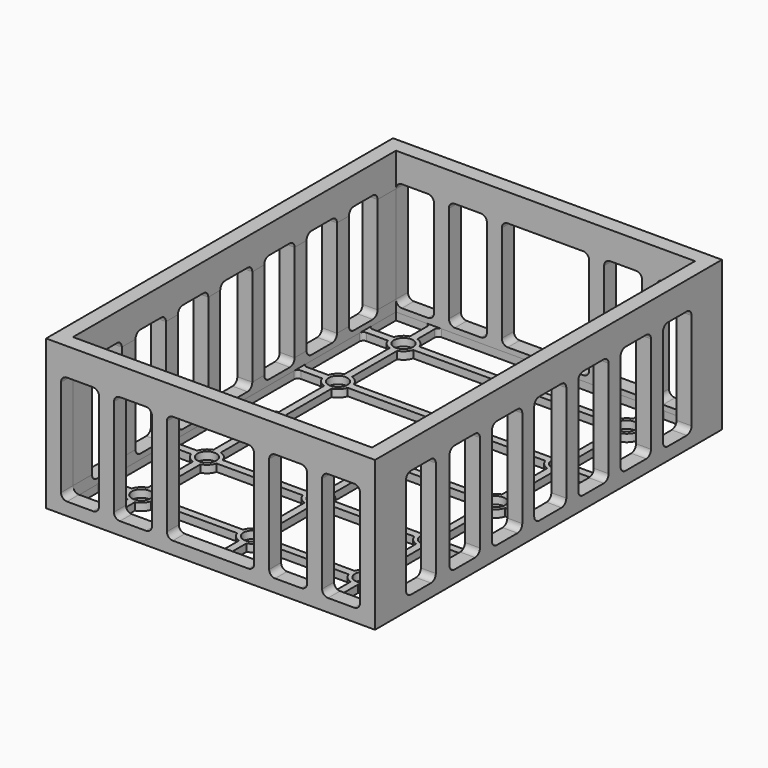
from build123d import *
from build123d import SkipClean  # not in build123d's __all__

# Parameters (mm, degrees)
F0_W      = 440
F0_H      = 580
F1_DEPTH  = 200
F2_W      = 400
F2_H      = 540
F3_DEPTH  = 190
F5_DEPTH  = 10
F4_R      = 12.7
F6_DEPTH  = 10
F8_DEPTH  = 440
F10_DEPTH = 580


# Not quite as in the source:
# - ends of sketch curves that miss each other by under 0.0002 mm in the source are joined


with BuildPart() as f1:
    # F0 (on Top) → F1 (new body)
    with BuildSketch(Plane.XY):
        with Locations((220, 290)):
            Rectangle(F0_W, F0_H)
    extrude(amount=F1_DEPTH)

    # F2 (on face) → F3 (cut)
    with BuildSketch(Plane.XY.offset(200)):
        with Locations((220, 290)):
            Rectangle(F2_W, F2_H)
    extrude(amount=-F3_DEPTH, mode=Mode.SUBTRACT)

    # F4 (on face) → F5 (cut, through all)
    with BuildSketch(Plane.XY.offset(10)):
        with BuildLine():
            ThreePointArc((53.8208951944, 514.2), (58.284209973, 521.715790027), (65.8, 526.1791048056))
            Line((65.8, 526.1791048056), (65.8, 555))
            ThreePointArc((65.8, 555), (64.3355339059, 558.5355339059), (60.8, 560))
            Line((60.8, 560), (20, 560))
            Line((20, 560), (20, 519.2))
            ThreePointArc((20, 519.2), (21.4644660941, 515.6644660941), (25, 514.2))
            Line((25, 514.2), (53.8208951944, 514.2))
        make_face()
        with BuildLine():
            ThreePointArc((75.8000016212, 526.1791043282), (83.3157906245, 521.7157894295), (87.7791048056, 514.2))
            Line((87.7791048056, 514.2), (203.0208951944, 514.2))
            ThreePointArc((203.0208951944, 514.2), (207.484209973, 521.715790027), (215, 526.1791048056))
            Line((215, 526.1791048056), (215, 555))
            ThreePointArc((215, 555), (213.5355339059, 558.5355339059), (210, 560))
            Line((210, 560), (80.8000016212, 560))
            ThreePointArc((80.8000016212, 560), (77.2644677153, 558.5355339059), (75.8000016212, 555))
            Line((75.8000016212, 555), (75.8000016212, 526.1791043282))
        make_face()
        with BuildLine():
            Line((225, 555), (225, 526.1791048056))
            ThreePointArc((225, 526.1791048056), (232.515790027, 521.715790027), (236.9791048056, 514.2))
            Line((236.9791048056, 514.2), (352.22089302, 514.2000006389))
            ThreePointArc((352.22089302, 514.2000006389), (356.684207757, 521.7157906907), (364.1999977593, 526.1791055109))
            Line((364.1999977593, 526.1791055109), (364.1999975996, 555.0000000277))
            ThreePointArc((364.1999975996, 555.0000000277), (362.7355314957, 558.5355339157), (359.1999975996, 560))
            Line((359.1999975996, 560), (230, 560))
            ThreePointArc((230, 560), (226.4644660941, 558.5355339059), (225, 555))
        make_face()
        with BuildLine():
            Line((419.9999978256, 560), (379.1999975996, 560))
            ThreePointArc((379.1999975996, 560), (375.6644636838, 558.5355338961), (374.1999975996, 554.9999999723))
            Line((374.1999975996, 554.9999999723), (374.1999977593, 526.1791055663))
            ThreePointArc((374.1999977593, 526.1791055663), (381.715787811, 521.7157908294), (386.1791026313, 514.2000008271))
            Line((386.1791026313, 514.2000008271), (414.9999978256, 514.2000009868))
            ThreePointArc((414.9999978256, 514.2000009868), (418.5355317316, 515.6644660941), (419.9999978256, 519.2))
            Line((419.9999978256, 519.2), (419.9999978256, 560))
        make_face()
        with BuildLine():
            Line((65.8, 416.5791048056), (65.8, 492.2208951944))
            ThreePointArc((65.8, 492.2208951944), (58.284209973, 496.684209973), (53.8208951944, 504.2))
            Line((53.8208951944, 504.2), (25, 504.2))
            ThreePointArc((25, 504.2), (21.4644660941, 502.7355339059), (20, 499.2))
            Line((20, 499.2), (20, 409.599994421))
            ThreePointArc((20, 409.599994421), (21.4644660941, 406.0644605151), (25, 404.599994421))
            Line((25, 404.599994421), (53.8208935515, 404.599994421))
            ThreePointArc((53.8208935515, 404.599994421), (58.2842079168, 412.1157879708), (65.8, 416.5791048056))
        make_face()
        with BuildLine():
            Line((203.0208951944, 504.2), (87.7791048056, 504.2))
            ThreePointArc((87.7791048056, 504.2), (83.3157906245, 496.6842105705), (75.8000016212, 492.2208956718))
            Line((75.8000016212, 492.2208956718), (75.8000016212, 416.5791043282))
            ThreePointArc((75.8000016212, 416.5791043282), (83.3157926808, 412.1157873732), (87.7791064485, 404.599994421))
            Line((87.7791064485, 404.599994421), (203.0208935515, 404.599994421))
            ThreePointArc((203.0208935515, 404.599994421), (207.4842079168, 412.1157879708), (215, 416.5791048056))
            Line((215, 416.5791048056), (215, 492.2208951944))
            ThreePointArc((215, 492.2208951944), (207.484209973, 496.684209973), (203.0208951944, 504.2))
        make_face()
        with BuildLine():
            ThreePointArc((236.9791048056, 504.2), (232.515790027, 496.684209973), (225, 492.2208951944))
            Line((225, 492.2208951944), (225, 416.5791048056))
            ThreePointArc((225, 416.5791048056), (232.5157920832, 412.1157879708), (236.9791064485, 404.599994421))
            Line((236.9791064485, 404.599994421), (352.2208919844, 404.5999950599))
            ThreePointArc((352.2208919844, 404.5999950599), (356.6842063081, 412.1157886344), (364.1999983666, 416.5791055109))
            Line((364.1999983666, 416.5791055109), (364.1999979474, 492.2208958997))
            ThreePointArc((364.1999979474, 492.2208958997), (356.6842078957, 496.6842106367), (352.2208930754, 504.2000006389))
            Line((352.2208930754, 504.2000006389), (236.9791048056, 504.2))
        make_face()
        with BuildLine():
            ThreePointArc((386.1791026867, 504.2000008271), (381.7157879497, 496.6842107754), (374.1999979474, 492.2208959551))
            Line((374.1999979474, 492.2208959551), (374.1999983666, 416.5791055663))
            ThreePointArc((374.1999983666, 416.5791055663), (381.7157904745, 412.1157887731), (386.1791048814, 404.5999952481))
            Line((386.1791048814, 404.5999952481), (414.9999984329, 404.5999954078))
            ThreePointArc((414.9999984329, 404.5999954078), (418.5355323389, 406.0644605151), (419.9999984329, 409.599994421))
            Line((419.9999984329, 409.599994421), (419.9999984329, 499.2))
            ThreePointArc((419.9999984329, 499.2), (418.5355323389, 502.7355339059), (414.9999984329, 504.2))
            Line((414.9999984329, 504.2), (386.1791026867, 504.2000008271))
        make_face()
        with BuildLine():
            ThreePointArc((65.8, 382.6208951944), (58.284209973, 387.084209973), (53.8208951944, 394.6))
            Line((53.8208951944, 394.6), (25, 394.6))
            ThreePointArc((25, 394.6), (21.4644660941, 393.1355339059), (20, 389.6))
            Line((20, 389.6), (20, 300))
            ThreePointArc((20, 300), (21.4644660941, 296.4644660941), (25, 295))
            Line((25, 295), (53.8208951944, 295))
            ThreePointArc((53.8208951944, 295), (58.284209973, 302.515790027), (65.8, 306.9791048056))
            Line((65.8, 306.9791048056), (65.8, 382.6208951944))
        make_face()
        with BuildLine():
            ThreePointArc((215, 382.6208951944), (207.484209973, 387.084209973), (203.0208951944, 394.6))
            Line((203.0208951944, 394.6), (87.7791048056, 394.6))
            ThreePointArc((87.7791048056, 394.6), (83.3157906245, 387.0842105705), (75.8000016212, 382.6208956718))
            Line((75.8000016212, 382.6208956718), (75.8000016212, 306.9791043282))
            ThreePointArc((75.8000016212, 306.9791043282), (83.3157906245, 302.5157894295), (87.7791048056, 295))
            Line((87.7791048056, 295), (203.0208951944, 295))
            ThreePointArc((203.0208951944, 295), (207.484209973, 302.515790027), (215, 306.9791048056))
            Line((215, 306.9791048056), (215, 382.6208951944))
        make_face()
        with BuildLine():
            ThreePointArc((236.9791048056, 394.6), (232.515790027, 387.084209973), (225, 382.6208951944))
            Line((225, 382.6208951944), (225, 306.9791048056))
            ThreePointArc((225, 306.9791048056), (232.515790027, 302.515790027), (236.9791048056, 295))
            Line((236.9791048056, 295), (352.2208942346, 295.0000006389))
            ThreePointArc((352.2208942346, 295.0000006389), (356.6842089716, 302.5157906907), (364.1999989738, 306.9791055109))
            Line((364.1999989738, 306.9791055109), (364.1999985547, 382.6208958997))
            ThreePointArc((364.1999985547, 382.6208958997), (356.684208503, 387.0842106367), (352.2208936827, 394.6000006389))
            Line((352.2208936827, 394.6000006389), (236.9791048056, 394.6))
        make_face()
        with BuildLine():
            ThreePointArc((386.179103294, 394.6000008271), (381.715788557, 387.0842107754), (374.1999985547, 382.6208959551))
            Line((374.1999985547, 382.6208959551), (374.1999989738, 306.9791055663))
            ThreePointArc((374.1999989738, 306.9791055663), (381.7157890256, 302.5157908294), (386.1791038458, 295.0000008271))
            Line((386.1791038458, 295.0000008271), (414.9999990402, 295.0000009868))
            ThreePointArc((414.9999990402, 295.0000009868), (418.535532957, 296.464466105), (419.9999990402, 300.0000000308))
            Line((419.9999990402, 300.0000000308), (419.9999984883, 389.6000000308))
            ThreePointArc((419.9999984883, 389.6000000308), (418.5355323834, 393.1355339168), (414.9999984883, 394.6))
            Line((414.9999984883, 394.6), (386.179103294, 394.6000008271))
        make_face()
        with BuildLine():
            ThreePointArc((25, 285), (21.4644660941, 283.5355339059), (20, 280))
            Line((20, 280), (20, 190.4))
            ThreePointArc((20, 190.4), (21.4644660941, 186.8644660941), (25, 185.4))
            Line((25, 185.4), (53.8208951944, 185.4))
            ThreePointArc((53.8208951944, 185.4), (58.284209973, 192.915790027), (65.8, 197.3791048056))
            Line((65.8, 197.3791048056), (65.8, 273.0208951944))
            ThreePointArc((65.8, 273.0208951944), (58.284209973, 277.484209973), (53.8208951944, 285))
            Line((53.8208951944, 285), (25, 285))
        make_face()
        with BuildLine():
            ThreePointArc((215, 273.0208951944), (207.484209973, 277.484209973), (203.0208951944, 285))
            Line((203.0208951944, 285), (87.7791048056, 285))
            ThreePointArc((87.7791048056, 285), (83.3157906245, 277.4842105705), (75.8000016212, 273.0208956718))
            Line((75.8000016212, 273.0208956718), (75.8000016212, 197.3791043282))
            ThreePointArc((75.8000016212, 197.3791043282), (83.3157906245, 192.9157894295), (87.7791048056, 185.4))
            Line((87.7791048056, 185.4), (203.0208951944, 185.4))
            ThreePointArc((203.0208951944, 185.4), (207.484209973, 192.915790027), (215, 197.3791048056))
            Line((215, 197.3791048056), (215, 273.0208951944))
        make_face()
        with BuildLine():
            Line((352.22089429, 285.0000006389), (236.9791048056, 285))
            ThreePointArc((236.9791048056, 285), (232.515790027, 277.484209973), (225, 273.0208951944))
            Line((225, 273.0208951944), (225, 197.3791048056))
            ThreePointArc((225, 197.3791048056), (232.515790027, 192.915790027), (236.9791048056, 185.4))
            Line((236.9791048056, 185.4), (352.2208953235, 185.4000008237))
            ThreePointArc((352.2208953235, 185.4000008237), (356.6842100813, 192.9157908631), (364.2000000959, 197.3791056625))
            Line((364.2000000959, 197.3791056625), (364.199999162, 273.0208958997))
            ThreePointArc((364.199999162, 273.0208958997), (356.6842091103, 277.4842106367), (352.22089429, 285.0000006389))
        make_face()
        with BuildLine():
            ThreePointArc((386.1791039012, 285.0000008271), (381.7157891643, 277.4842107754), (374.199999162, 273.0208959551))
            Line((374.199999162, 273.0208959551), (374.1999995811, 197.3791058418))
            ThreePointArc((374.1999995811, 197.3791058418), (381.7157899456, 192.9157911222), (386.1791049347, 185.4000009178))
            Line((386.1791049347, 185.4000009178), (415.0000001291, 185.4000009976))
            ThreePointArc((415.0000001291, 185.4000009976), (418.5355340554, 186.8644661145), (420.0000001291, 190.4000000577))
            Line((420.0000001291, 190.4000000577), (419.9999990956, 280.0000000577))
            ThreePointArc((419.9999990956, 280.0000000577), (418.5355329812, 283.5355339263), (414.9999990956, 285))
            Line((414.9999990956, 285), (386.1791039012, 285.0000008271))
        make_face()
        with BuildLine():
            ThreePointArc((25, 175.4), (21.4644660941, 173.9355339059), (20, 170.4))
            Line((20, 170.4), (20, 80.8000016212))
            ThreePointArc((20, 80.8000016212), (21.4644660941, 77.2644677153), (25, 75.8000016212))
            Line((25, 75.8000016212), (53.8208956718, 75.8000016212))
            ThreePointArc((53.8208956718, 75.8000016212), (58.2842105705, 83.3157906245), (65.8, 87.7791048056))
            Line((65.8, 87.7791048056), (65.8, 163.4208951944))
            ThreePointArc((65.8, 163.4208951944), (58.284209973, 167.884209973), (53.8208951944, 175.4))
            Line((53.8208951944, 175.4), (25, 175.4))
        make_face()
        with BuildLine():
            ThreePointArc((215, 163.4208951944), (207.484209973, 167.884209973), (203.0208951944, 175.4))
            Line((203.0208951944, 175.4), (87.7791048056, 175.4))
            ThreePointArc((87.7791048056, 175.4), (83.3157906245, 167.8842105705), (75.8000016212, 163.4208956718))
            Line((75.8000016212, 163.4208956718), (75.8000016212, 87.7791043282))
            ThreePointArc((75.8000016212, 87.7791043282), (83.315790027, 83.315790027), (87.7791043282, 75.8000016212))
            Line((87.7791043282, 75.8000016212), (203.0208956718, 75.8000016212))
            ThreePointArc((203.0208956718, 75.8000016212), (207.4842105705, 83.3157906245), (215, 87.7791048056))
            Line((215, 87.7791048056), (215, 163.4208951944))
        make_face()
        with BuildLine():
            ThreePointArc((364.2000003472, 163.420896005), (356.6842102086, 167.8842107512), (352.2208953512, 175.4000008237))
            Line((352.2208953512, 175.4000008237), (236.9791048056, 175.4))
            ThreePointArc((236.9791048056, 175.4), (232.515790027, 167.884209973), (225, 163.4208951944))
            Line((225, 163.4208951944), (225, 87.7791048056))
            ThreePointArc((225, 87.7791048056), (232.5157894295, 83.3157906245), (236.9791043282, 75.8000016212))
            Line((236.9791043282, 75.8000016212), (352.2208956718, 75.8000016212))
            ThreePointArc((352.2208956718, 75.8000016212), (356.6842105454, 83.31579121), (364.2000003472, 87.7791057247))
            Line((364.2000003472, 87.7791057247), (364.2000003472, 163.420896005))
        make_face()
        with BuildLine():
            Line((420.0000001568, 80.8000016212), (420.0000001568, 170.4))
            ThreePointArc((420.0000001568, 170.4), (418.5355340628, 173.9355339059), (415.0000001568, 175.4))
            Line((415.0000001568, 175.4), (386.1791049624, 175.4000009178))
            ThreePointArc((386.1791049624, 175.4000009178), (381.7157900496, 167.8842107234), (374.1999997693, 163.4208959551))
            Line((374.1999997693, 163.4208959551), (374.2000001884, 87.7791057715))
            ThreePointArc((374.2000001884, 87.7791057715), (381.7157900905, 83.3157912685), (386.1791050226, 75.8000016212))
            Line((386.1791050226, 75.8000016212), (415.0000001568, 75.8000016212))
            ThreePointArc((415.0000001568, 75.8000016212), (418.5355340628, 77.2644677153), (420.0000001568, 80.8000016212))
        make_face()
        with BuildLine():
            ThreePointArc((25, 65.8), (21.4644660941, 64.3355339059), (20, 60.8))
            Line((20, 60.8), (20, 20))
            Line((20, 20), (65.8, 20))
            Line((65.8, 20), (65.8, 53.8208951944))
            ThreePointArc((65.8, 53.8208951944), (58.284209973, 58.284209973), (53.8208951944, 65.8))
            Line((53.8208951944, 65.8), (25, 65.8))
        make_face()
        with BuildLine():
            Line((75.8000016212, 53.8208956718), (75.8000016212, 20))
            Line((75.8000016212, 20), (215, 20))
            Line((215, 20), (215, 53.8208951944))
            ThreePointArc((215, 53.8208951944), (207.484209973, 58.284209973), (203.0208951944, 65.8))
            Line((203.0208951944, 65.8), (87.7791048056, 65.8))
            ThreePointArc((87.7791048056, 65.8), (83.3157906245, 58.2842105705), (75.8000016212, 53.8208956718))
        make_face()
        with BuildLine():
            Line((225, 53.8208951944), (225, 20))
            Line((225, 20), (364.2000003472, 20))
            Line((364.2000003472, 20), (364.2000003472, 53.8208958965))
            ThreePointArc((364.2000003472, 53.8208958965), (356.6842105454, 58.2842104113), (352.2208956718, 65.8))
            Line((352.2208956718, 65.8), (236.9791048056, 65.8))
            ThreePointArc((236.9791048056, 65.8), (232.515790027, 58.284209973), (225, 53.8208951944))
        make_face()
        with BuildLine():
            Line((420, 20), (420, 60.8))
            ThreePointArc((420, 60.8), (418.5355339059, 64.3355339059), (415, 65.8))
            Line((415, 65.8), (386.1791050226, 65.8))
            ThreePointArc((386.1791050226, 65.8), (381.7157901598, 58.2842104221), (374.2000003766, 53.8208959052))
            Line((374.2000003766, 53.8208959052), (374.200000564, 20.0000007607))
            Line((374.200000564, 20.0000007607), (420, 20))
        make_face()
    with SkipClean():  # cleaning this boolean's faces spoils the solid; the shape is the same uncleaned
        extrude(amount=-F5_DEPTH, mode=Mode.SUBTRACT)

    # F4 (on face) → F6 (cut, through all)
    with BuildSketch(Plane.XY.offset(10)):
        with Locations((70.8, 509.2)):
            Circle(F4_R)
        with Locations((70.8, 399.6)):
            Circle(F4_R)
        with Locations((70.8, 290)):
            Circle(F4_R)
        with Locations((70.8, 180.4)):
            Circle(F4_R)
        with Locations((70.8, 70.8)):
            Circle(F4_R)
        with Locations((220, 509.2)):
            Circle(F4_R)
        with Locations((220, 399.6)):
            Circle(F4_R)
        with Locations((220, 290)):
            Circle(F4_R)
        with Locations((220, 180.4)):
            Circle(F4_R)
        with Locations((220, 70.8)):
            Circle(F4_R)
        with Locations((369.2000003472, 70.8000008106)):
            Circle(F4_R)
        with Locations((369.200000143, 180.4000008708)):
            Circle(F4_R)
        with Locations((369.1999990679, 290.000000733)):
            Circle(F4_R)
        with Locations((369.1999984606, 399.600000733)):
            Circle(F4_R)
        with Locations((369.1999978534, 509.200000733)):
            Circle(F4_R)
    with SkipClean():  # cleaning this boolean's faces spoils the solid; the shape is the same uncleaned
        extrude(amount=-F6_DEPTH, mode=Mode.SUBTRACT)

    # F7 (on face) → F8 (cut, through all)
    with BuildSketch(Plane.YZ.offset(440)):
        with BuildLine():
            ThreePointArc((51.7702624202, 25), (54.1134081707, 19.3431457505), (59.7702624202, 17))
            Line((59.7702624202, 17), (93.6, 17))
            ThreePointArc((93.6, 17), (99.2568542495, 19.3431457505), (101.6, 25))
            Line((101.6, 25), (101.6, 155))
            ThreePointArc((101.6, 155), (99.2568542495, 160.6568542495), (93.6, 163))
            Line((93.6, 163), (59.7702624202, 163))
            ThreePointArc((59.7702624202, 163), (54.1134081707, 160.6568542495), (51.7702624202, 155))
            Line((51.7702624202, 155), (51.7702624202, 25))
        make_face()
        with BuildLine():
            Line((124.6, 155), (124.6, 25))
            ThreePointArc((124.6, 25), (126.9431457505, 19.3431457505), (132.6, 17))
            Line((132.6, 17), (167.4, 17))
            ThreePointArc((167.4, 17), (173.0568542495, 19.3431457505), (175.4, 25))
            Line((175.4, 25), (175.4, 155))
            ThreePointArc((175.4, 155), (173.0568542495, 160.6568542495), (167.4, 163))
            Line((167.4, 163), (132.6, 163))
            ThreePointArc((132.6, 163), (126.9431457505, 160.6568542495), (124.6, 155))
        make_face()
        with BuildLine():
            Line((195.4, 155), (195.4, 25))
            ThreePointArc((195.4, 25), (197.7431457505, 19.3431457505), (203.4, 17))
            Line((203.4, 17), (238.2, 17))
            ThreePointArc((238.2, 17), (243.8568542495, 19.3431457505), (246.2, 25))
            Line((246.2, 25), (246.2, 155))
            ThreePointArc((246.2, 155), (243.8568542495, 160.6568542495), (238.2, 163))
            Line((238.2, 163), (203.4, 163))
            ThreePointArc((203.4, 163), (197.7431457505, 160.6568542495), (195.4, 155))
        make_face()
        with BuildLine():
            Line((266.2, 155), (266.2, 25))
            ThreePointArc((266.2, 25), (268.5431457505, 19.3431457505), (274.2, 17))
            Line((274.2, 17), (311.8, 17))
            ThreePointArc((311.8, 17), (317.4568542495, 19.3431457505), (319.8, 25))
            Line((319.8, 25), (319.8, 155))
            ThreePointArc((319.8, 155), (317.4568542495, 160.6568542495), (311.8, 163))
            Line((311.8, 163), (274.2, 163))
            ThreePointArc((274.2, 163), (268.5431457505, 160.6568542495), (266.2, 155))
        make_face()
        with BuildLine():
            ThreePointArc((382.6, 17), (388.2568542495, 19.3431457505), (390.6, 25))
            Line((390.6, 25), (390.6, 155))
            ThreePointArc((390.6, 155), (388.2568542495, 160.6568542495), (382.6, 163))
            Line((382.6, 163), (347.8, 163))
            ThreePointArc((347.8, 163), (342.1431457505, 160.6568542495), (339.8, 155))
            Line((339.8, 155), (339.8, 25))
            ThreePointArc((339.8, 25), (342.1431457505, 19.3431457505), (347.8, 17))
            Line((347.8, 17), (382.6, 17))
        make_face()
        with BuildLine():
            ThreePointArc((453.4, 17), (459.0568542495, 19.3431457505), (461.4, 25))
            Line((461.4, 25), (461.4, 155))
            ThreePointArc((461.4, 155), (459.0568542495, 160.6568542495), (453.4, 163))
            Line((453.4, 163), (418.6, 163))
            ThreePointArc((418.6, 163), (412.9431457505, 160.6568542495), (410.6, 155))
            Line((410.6, 155), (410.6, 25))
            ThreePointArc((410.6, 25), (412.9431457505, 19.3431457505), (418.6, 17))
            Line((418.6, 17), (453.4, 17))
        make_face()
        with BuildLine():
            ThreePointArc((521.2, 17), (526.8568542495, 19.3431457505), (529.2, 25))
            Line((529.2, 25), (529.2, 155))
            ThreePointArc((529.2, 155), (526.8568542495, 160.6568542495), (521.2, 163))
            Line((521.2, 163), (489.4, 163))
            ThreePointArc((489.4, 163), (483.7431457505, 160.6568542495), (481.4, 155))
            Line((481.4, 155), (481.4, 25))
            ThreePointArc((481.4, 25), (483.7431457505, 19.3431457505), (489.4, 17))
            Line((489.4, 17), (521.2, 17))
        make_face()
    with SkipClean():  # cleaning this boolean's faces spoils the solid; the shape is the same uncleaned
        extrude(amount=-F8_DEPTH, mode=Mode.SUBTRACT)

    # F9 (on face) → F10 (cut, through all)
    with BuildSketch(Plane.XZ):
        with BuildLine():
            Line((20, 155), (20, 25))
            ThreePointArc((20, 25), (22.3431457505, 19.3431457505), (28, 17))
            Line((28, 17), (62.8, 17))
            ThreePointArc((62.8, 17), (68.4568542495, 19.3431457505), (70.8, 25))
            Line((70.8, 25), (70.8, 155))
            ThreePointArc((70.8, 155), (68.4568542495, 160.6568542495), (62.8, 163))
            Line((62.8, 163), (28, 163))
            ThreePointArc((28, 163), (22.3431457505, 160.6568542495), (20, 155))
        make_face()
        with BuildLine():
            Line((90.8, 155), (90.8, 25))
            ThreePointArc((90.8, 25), (93.1431457505, 19.3431457505), (98.8, 17))
            Line((98.8, 17), (133.6, 17))
            ThreePointArc((133.6, 17), (139.2568542495, 19.3431457505), (141.6, 25))
            Line((141.6, 25), (141.6, 155))
            ThreePointArc((141.6, 155), (139.2568542495, 160.6568542495), (133.6, 163))
            Line((133.6, 163), (98.8, 163))
            ThreePointArc((98.8, 163), (93.1431457505, 160.6568542495), (90.8, 155))
        make_face()
        with BuildLine():
            Line((161.6, 155), (161.6, 25))
            ThreePointArc((161.6, 25), (163.9431457505, 19.3431457505), (169.6, 17))
            Line((169.6, 17), (270.4, 17))
            ThreePointArc((270.4, 17), (276.0568542495, 19.3431457505), (278.4, 25))
            Line((278.4, 25), (278.4, 155))
            ThreePointArc((278.4, 155), (276.0568542495, 160.6568542495), (270.4, 163))
            Line((270.4, 163), (169.6, 163))
            ThreePointArc((169.6, 163), (163.9431457505, 160.6568542495), (161.6, 155))
        make_face()
        with BuildLine():
            ThreePointArc((341.2, 17), (346.8568542495, 19.3431457505), (349.2, 25))
            Line((349.2, 25), (349.2, 155))
            ThreePointArc((349.2, 155), (346.8568542495, 160.6568542495), (341.2, 163))
            Line((341.2, 163), (306.4, 163))
            ThreePointArc((306.4, 163), (300.7431457505, 160.6568542495), (298.4, 155))
            Line((298.4, 155), (298.4, 25))
            ThreePointArc((298.4, 25), (300.7431457505, 19.3431457505), (306.4, 17))
            Line((306.4, 17), (341.2, 17))
        make_face()
        with BuildLine():
            ThreePointArc((412, 17), (417.6568542495, 19.3431457505), (420, 25))
            Line((420, 25), (420, 155))
            ThreePointArc((420, 155), (417.6568542495, 160.6568542495), (412, 163))
            Line((412, 163), (377.2, 163))
            ThreePointArc((377.2, 163), (371.5431457505, 160.6568542495), (369.2, 155))
            Line((369.2, 155), (369.2, 25))
            ThreePointArc((369.2, 25), (371.5431457505, 19.3431457505), (377.2, 17))
            Line((377.2, 17), (412, 17))
        make_face()
    with SkipClean():  # cleaning this boolean's faces spoils the solid; the shape is the same uncleaned
        extrude(amount=-F10_DEPTH, mode=Mode.SUBTRACT)


with BuildPart() as f11_1:
    # F11: copy of F1
    add(f1.part, clean=False)


solid = f1.part
